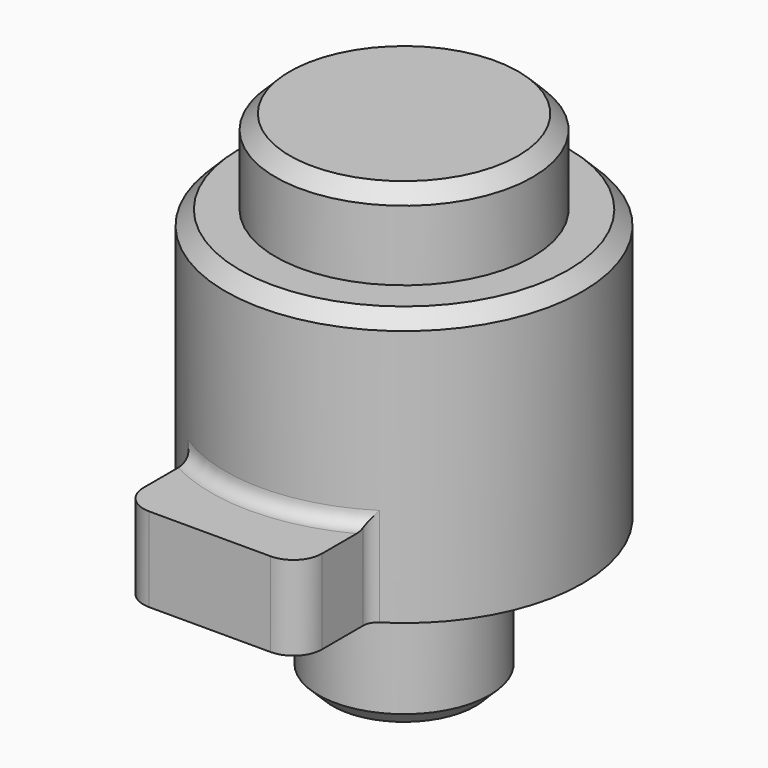
from build123d import *

# Parameters (mm, degrees)
F0_R     = 2.286
F1_DEPTH = 1.5
F2_R     = 3.175
F2_R_2   = 2.286
F3_DEPTH = 4.826
F4_SIZE  = 0.254
F5_R     = 1.524
F6_DEPTH = 2.54
F7_W     = 3.175
F7_H     = 1.5
F8_DEPTH = 4.318
F9_R     = 0.508
F10_SIZE = 0.254
F11_R    = 0.254
F12_SIZE = 0.254


# Not quite as in the source:
# - a feature names something its author has since deleted; it is built from what else it names


with BuildPart() as f1:
    # F0 (on Top) → F1 (new body)
    with BuildSketch(Plane.XY):
        Circle(F0_R)
    extrude(amount=F1_DEPTH)

    # F2 (on face) → F3 (join)
    with BuildSketch(Plane(origin=(0, 0, 0), x_dir=(1, 0, 0), z_dir=(0, 0, -1))):
        Circle(F2_R)
        Circle(F2_R_2, mode=Mode.SUBTRACT)
        Circle(F2_R_2)
    extrude(amount=F3_DEPTH)

    # F4
    f4_edges = [f1.edges().sort_by_distance(p)[0] for p in [
        (-2.286, 0, 1.5),
    ]]
    chamfer(f4_edges, length=F4_SIZE)

    # F5 (on face) → F6 (join)
    with BuildSketch(Plane(origin=(0, 0, -4.826), x_dir=(1, 0, 0), z_dir=(0, 0, -1))):
        Circle(F5_R)
    extrude(amount=F6_DEPTH)

    # F7 (on Front) → F8 (join)
    with BuildSketch(Plane.XZ):
        with Locations((0, -4.076)):
            Rectangle(F7_W, F7_H)
    extrude(amount=F8_DEPTH)

    # F9
    f9_edges = [f1.edges().sort_by_distance(p)[0] for p in [
        (-1.5875, -4.318, -4.076),
        (1.5875, -4.318, -4.076),
    ]]
    fillet(f9_edges, radius=F9_R)

    # F10
    f10_edges = [f1.edges().sort_by_distance(p)[0] for p in [
        (-1.524, 0, -7.366),
    ]]
    chamfer(f10_edges, length=F10_SIZE)

    # F11
    f11_edges = [f1.edges().sort_by_distance(p)[0] for p in [
        (0, -3.175, -3.326),
        (1.5875, -2.749631, -4.076),
        (-1.5875, -2.749631, -4.076),
    ]]
    fillet(f11_edges, radius=F11_R)

    # F12
    f12_edges = [f1.edges().sort_by_distance(p)[0] for p in [
        (-3.175, 0, 0),
    ]]
    chamfer(f12_edges, length=F12_SIZE)


solid = f1.part
